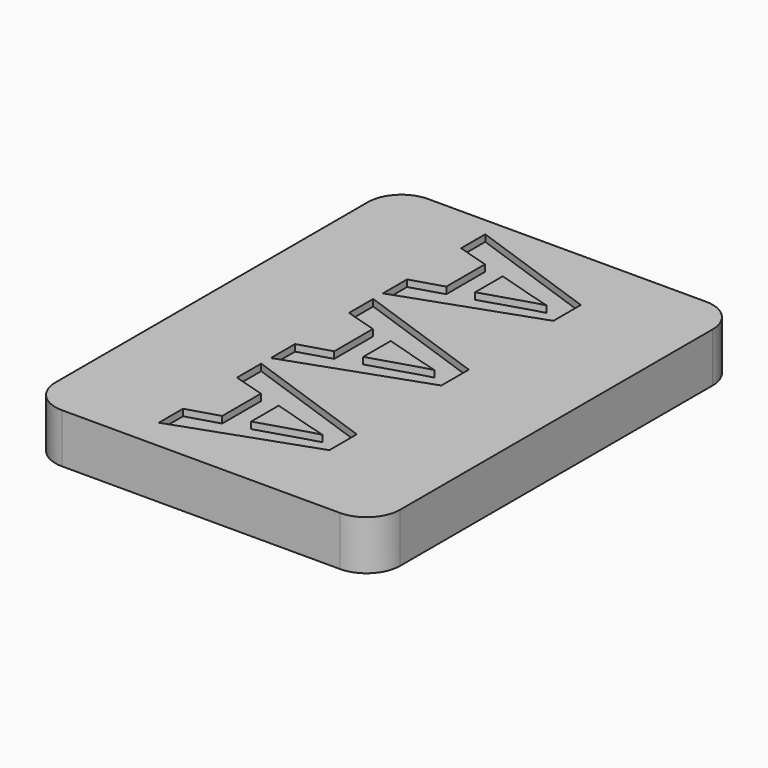
from build123d import *

# Parameters (mm, degrees)
F0_W          = 65.532
F0_H          = 86.995
F1_DEPTH      = 41.275
F2_R          = 5.3975
F3_DEPTH      = 38.1
F4_R          = 6.35
F6_DEPTH      = 6.858
F8_DEPTH      = 2.54
F10_TEXT_SIZE = 35.2777777778
F11_DEPTH     = 1.27


# Not quite as in the source:
# - Text() gives the source's letters only with a copy of the font that has no kerning and outlines rounded to 1/6400 em; it was checked with that copy


with BuildPart() as f1:
    # F0 (on Top) → F1 (new body)
    with BuildSketch(Plane.XY):
        Rectangle(F0_W, F0_H)
    extrude(amount=F1_DEPTH)

    # F2 (on face) → F3 (cut)
    with BuildSketch(Plane.XY.offset(41.275)):
        with Locations((-24.1935, 34.925)):
            Circle(F2_R)
        with Locations((-24.1935, 20.955)):
            Circle(F2_R)
        with Locations((-24.1935, 6.985)):
            Circle(F2_R)
        with Locations((-24.1935, -6.985)):
            Circle(F2_R)
        with Locations((-24.1935, -20.955)):
            Circle(F2_R)
        with Locations((-24.1935, -34.925)):
            Circle(F2_R)
        with Locations((-12.0951251091, 27.94)):
            Circle(F2_R)
        with Locations((-12.0951251091, 13.97)):
            Circle(F2_R)
        with Locations((-12.0951251091, 0)):
            Circle(F2_R)
        with Locations((-12.0951251091, -13.97)):
            Circle(F2_R)
        with Locations((-12.0951251091, -27.94)):
            Circle(F2_R)
        with Locations((12.1016246726, 0)):
            Circle(F2_R)
        with Locations((12.1016246726, 13.97)):
            Circle(F2_R)
        with Locations((12.1016246726, -13.97)):
            Circle(F2_R)
        with Locations((0.0032497817, 6.985)):
            Circle(F2_R)
        with Locations((0.0032497817, 20.955)):
            Circle(F2_R)
        with Locations((0.0032497817, 34.925)):
            Circle(F2_R)
        with Locations((12.1016246726, -27.94)):
            Circle(F2_R)
        with Locations((12.1016246726, 27.94)):
            Circle(F2_R)
        with Locations((0.0032497817, -6.985)):
            Circle(F2_R)
        with Locations((0.0032497817, -20.955)):
            Circle(F2_R)
        with Locations((0.0032497817, -34.925)):
            Circle(F2_R)
        with Locations((24.1999995635, 6.985)):
            Circle(F2_R)
        with Locations((24.1999995635, 20.955)):
            Circle(F2_R)
        with Locations((24.1999995635, 34.925)):
            Circle(F2_R)
        with Locations((24.1999995635, -6.985)):
            Circle(F2_R)
        with Locations((24.1999995635, -20.955)):
            Circle(F2_R)
        with Locations((24.1999995635, -34.925)):
            Circle(F2_R)
    extrude(amount=-F3_DEPTH, mode=Mode.SUBTRACT)

    # F4
    f4_edges = [f1.edges().sort_by_distance(p)[0] for p in [
        (-32.766, -43.4975, 20.6375),
        (32.766, -43.4975, 20.6375),
        (32.766, 43.4975, 20.6375),
        (-32.766, 43.4975, 20.6375),
    ]]
    fillet(f4_edges, radius=F4_R)


with BuildPart() as f6:
    # F5 (on face) → F6 (new body)
    with BuildSketch(Plane.XY.offset(41.275)):
        with BuildLine():
            Line((26.416, 43.4975), (-26.416, 43.4975))
            ThreePointArc((-26.416, 43.4975), (-30.9061280605, 41.6376280605), (-32.766, 37.1475))
            Line((-32.766, 37.1475), (-32.766, -37.1475))
            ThreePointArc((-32.766, -37.1475), (-30.9061280605, -41.6376280605), (-26.416, -43.4975))
            Line((-26.416, -43.4975), (26.416, -43.4975))
            ThreePointArc((26.416, -43.4975), (30.9061280605, -41.6376280605), (32.766, -37.1475))
            Line((32.766, -37.1475), (32.766, 37.1475))
            ThreePointArc((32.766, 37.1475), (30.9061280605, 41.6376280605), (26.416, 43.4975))
        make_face()
        with BuildLine():
            ThreePointArc((23.368, 40.4495), (27.8581280605, 38.5896280605), (29.718, 34.0995))
            Line((29.718, 34.0995), (29.718, -34.0995))
            ThreePointArc((29.718, -34.0995), (27.8581280605, -38.5896280605), (23.368, -40.4495))
            Line((23.368, -40.4495), (-23.368, -40.4495))
            ThreePointArc((-23.368, -40.4495), (-27.8581280605, -38.5896280605), (-29.718, -34.0995))
            Line((-29.718, -34.0995), (-29.718, 34.0995))
            ThreePointArc((-29.718, 34.0995), (-27.8581280605, 38.5896280605), (-23.368, 40.4495))
            Line((-23.368, 40.4495), (23.368, 40.4495))
        make_face(mode=Mode.SUBTRACT)
    extrude(amount=F6_DEPTH)

    # F7 (on face) → F8 (join)
    with BuildSketch(Plane.XY.offset(48.133)):
        with BuildLine():
            ThreePointArc((-26.416, 43.4975), (-30.9061280605, 41.6376280605), (-32.766, 37.1475))
            Line((-32.766, 37.1475), (-32.766, -37.1475))
            ThreePointArc((-32.766, -37.1475), (-30.9061280605, -41.6376280605), (-26.416, -43.4975))
            Line((-26.416, -43.4975), (26.416, -43.4975))
            ThreePointArc((26.416, -43.4975), (30.9061280605, -41.6376280605), (32.766, -37.1475))
            Line((32.766, -37.1475), (32.766, 37.1475))
            ThreePointArc((32.766, 37.1475), (30.9061280605, 41.6376280605), (26.416, 43.4975))
            Line((26.416, 43.4975), (-26.416, 43.4975))
        make_face()
    extrude(amount=F8_DEPTH)

    # F10 (on face) → F11 (cut)
    with BuildSketch(Plane.XY.offset(50.673)):
        with Locations(Location((-12.7, 39.9438151042), (0, 0, -90))):
            Text('A', F10_TEXT_SIZE, font='Open Sans', font_style=FontStyle.BOLD, text_align=(TextAlign.LEFT, TextAlign.BOTTOM))
        with Locations(Location((-12.7, 13.3146050347), (0, 0, -90))):
            Text('A', F10_TEXT_SIZE, font='Open Sans', font_style=FontStyle.BOLD, text_align=(TextAlign.LEFT, TextAlign.BOTTOM))
        with Locations(Location((-12.7, -13.3146050347), (0, 0, -90))):
            Text('A', F10_TEXT_SIZE, font='Open Sans', font_style=FontStyle.BOLD, text_align=(TextAlign.LEFT, TextAlign.BOTTOM))
    extrude(amount=-F11_DEPTH, mode=Mode.SUBTRACT)


solid = f6.part
